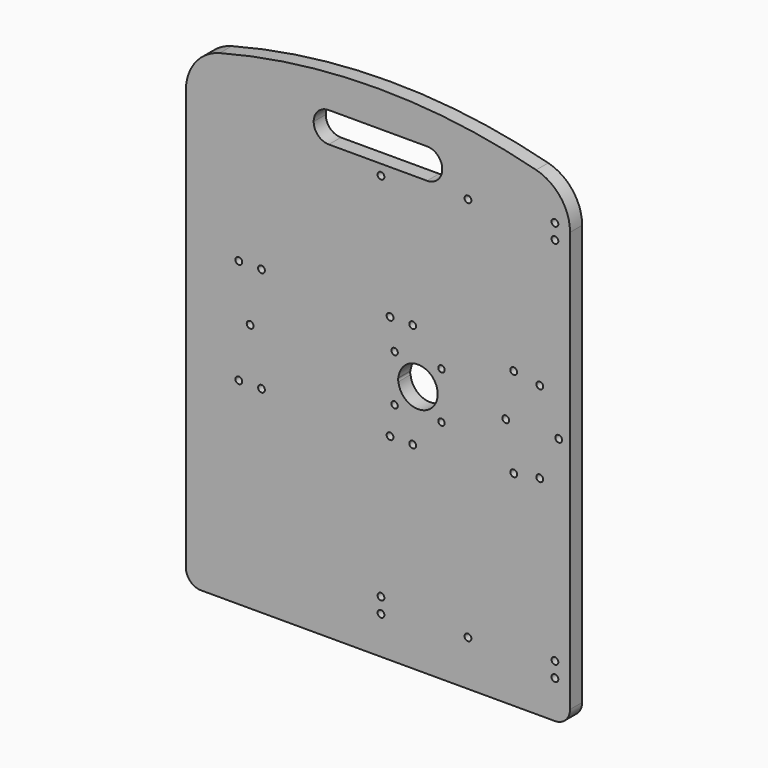
from build123d import *

# Parameters (mm, degrees)
F0_R     = 2.25
F0_R_2   = 2.125
F0_W     = 85
F0_H     = 20
F1_DEPTH = 5
F2_R     = 9.99999
F3_R     = 30


# Not quite as in the source:
# - a fillet or chamfer is up to 0.001 mm smaller than in the source, because OpenCascade refuses the exact size


with BuildPart() as f1:
    # F0 (on Front) → F1 (new body, symmetric)
    with BuildSketch(Plane.XZ):
        with BuildLine():
            Line((-127, -165.1), (127, -165.1))
            Line((127, -165.1), (127, 145.1))
            ThreePointArc((127, 145.1), (0, 165.1), (-127, 145.1))
            Line((-127, 145.1), (-127, -165.1))
        make_face()
        with Locations((-92, -34.75)):
            Circle(F0_R, mode=Mode.SUBTRACT)
        with Locations((-77, -34.75)):
            Circle(F0_R, mode=Mode.SUBTRACT)
        with Locations((-84.5, 0)):
            Circle(F0_R, mode=Mode.SUBTRACT)
        with Locations((2, -140.1)):
            Circle(F0_R, mode=Mode.SUBTRACT)
        with Locations((2, -130.1)):
            Circle(F0_R, mode=Mode.SUBTRACT)
        with Locations((59.5, -135.1)):
            Circle(F0_R, mode=Mode.SUBTRACT)
        with Locations((117, -140.1)):
            Circle(F0_R, mode=Mode.SUBTRACT)
        with Locations((117, -130.1)):
            Circle(F0_R, mode=Mode.SUBTRACT)
        with Locations((8, -34.75)):
            Circle(F0_R, mode=Mode.SUBTRACT)
        with Locations((23, -34.75)):
            Circle(F0_R, mode=Mode.SUBTRACT)
        with Locations((11, -15.5)):
            Circle(F0_R_2, mode=Mode.SUBTRACT)
        with BuildLine():
            ThreePointArc((13.5482954545, -1.1195308693), (13.25, 0), (13.5482954545, 1.1195308693))
            ThreePointArc((13.5482954545, 1.1195308693), (27.0602860471, 12.9879205243), (39.5, 0))
            ThreePointArc((39.5, 0), (27.0602860471, -12.9879205243), (13.5482954545, -1.1195308693))
        make_face(mode=Mode.SUBTRACT)
        with Locations((42, -15.5)):
            Circle(F0_R_2, mode=Mode.SUBTRACT)
        with Locations((89.75, -29.75)):
            Circle(F0_R, mode=Mode.SUBTRACT)
        with Locations((84.5, 0)):
            Circle(F0_R, mode=Mode.SUBTRACT)
        with Locations((107, -27)):
            Circle(F0_R, mode=Mode.SUBTRACT)
        with Locations((119.5, 0)):
            Circle(F0_R, mode=Mode.SUBTRACT)
        with Locations((-92, 34.75)):
            Circle(F0_R, mode=Mode.SUBTRACT)
        with Locations((-77, 34.75)):
            Circle(F0_R, mode=Mode.SUBTRACT)
        with Locations((11, 15.5)):
            Circle(F0_R_2, mode=Mode.SUBTRACT)
        with Locations((8, 34.75)):
            Circle(F0_R, mode=Mode.SUBTRACT)
        with Locations((23, 34.75)):
            Circle(F0_R, mode=Mode.SUBTRACT)
        with Locations((42, 15.5)):
            Circle(F0_R_2, mode=Mode.SUBTRACT)
        with Locations((89.75, 29.75)):
            Circle(F0_R, mode=Mode.SUBTRACT)
        with Locations((107, 27)):
            Circle(F0_R, mode=Mode.SUBTRACT)
        with Locations((2, 114.9)):
            Circle(F0_R, mode=Mode.SUBTRACT)
        with Locations((59.5, 119.9)):
            Circle(F0_R, mode=Mode.SUBTRACT)
        with Locations((0, 131.9)):
            Rectangle(F0_W, F0_H, mode=Mode.SUBTRACT)
        with Locations((117, 114.9)):
            Circle(F0_R, mode=Mode.SUBTRACT)
        with Locations((117, 124.9)):
            Circle(F0_R, mode=Mode.SUBTRACT)
    extrude(amount=F1_DEPTH, both=True)

    # F2 (radius 10 in the source; OpenCascade refuses exactly that, so slightly less here)
    f2_edges = [f1.edges().sort_by_distance(p)[0] for p in [
        (-127, 0, -165.1),
        (127, 0, -165.1),
        (-42.5, 0, 141.9),
        (-42.5, 0, 121.9),
        (42.5, 0, 141.9),
        (42.5, 0, 121.9),
    ]]
    fillet(f2_edges, radius=F2_R)

    # F3
    f3_edges = [f1.edges().sort_by_distance(p)[0] for p in [
        (127, 0, 145.1),
        (-127, 0, 145.1),
    ]]
    fillet(f3_edges, radius=F3_R)


solid = f1.part
